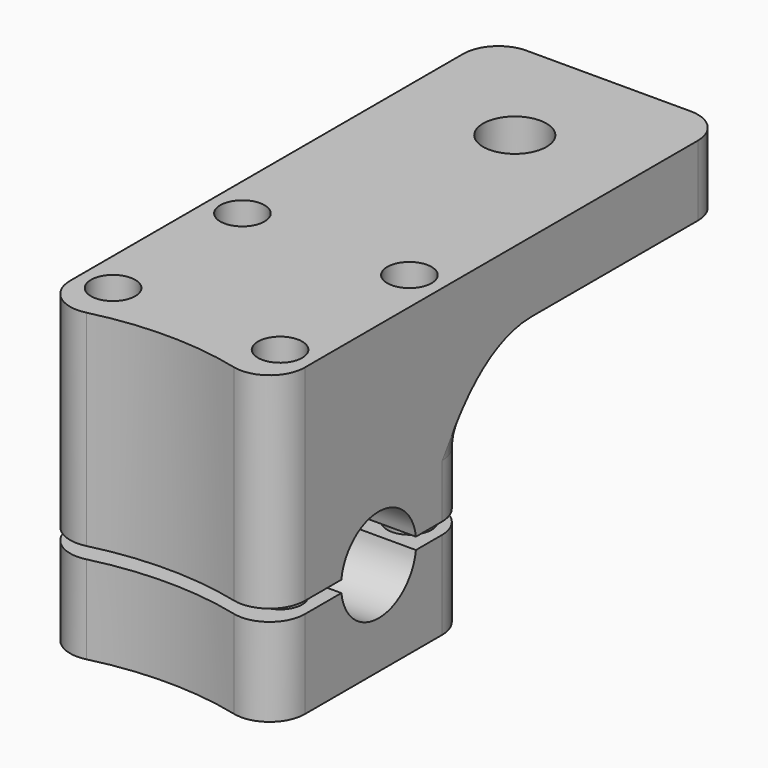
from build123d import *

# Parameters (mm, degrees)
F0_W         = 20
F0_H         = 22.7722101178
F0_R         = 1.8861050589
F0_H_2       = 26.2277898822
F0_R_2       = 2.7
F1_DEPTH     = 6
F2_DEPTH     = 20
F4_DEPTH     = 20.001
F6_DEPTH     = 20
F7_DEPTH     = 26.001
F8_R         = 3
F9_T2_ANGLE  = 25.7767353783
F9_T6_ANGLE  = 359.64
F9_T11_ANGLE = 359.64
F10_DEPTH    = 20.0010001


# Not quite as in the source:
# - a fillet or chamfer that OpenCascade refuses, or shapes differently, is made with other operations: its cross-section is extruded or revolved along the edge and cut away or added


with BuildPart() as f1:
    # F0 (on Top) → F1 (new body)
    with BuildSketch(Plane.XY):
        with Locations((0, -13.1138949411)):
            Rectangle(F0_W, F0_H)
        with Locations((-7.1138949411, -19.3861050589)):
            Circle(F0_R, mode=Mode.SUBTRACT)
        with Locations((-7.1138949411, -5.6138949411)):
            Circle(F0_R, mode=Mode.SUBTRACT)
        with Locations((7.1138949411, -19.3861050589)):
            Circle(F0_R, mode=Mode.SUBTRACT)
        with Locations((7.1138949411, -5.6138949411)):
            Circle(F0_R, mode=Mode.SUBTRACT)
        with Locations((0, 11.3861050589)):
            Rectangle(F0_W, F0_H_2)
        with Locations((0, 14.5)):
            Circle(F0_R_2, mode=Mode.SUBTRACT)
    extrude(amount=F1_DEPTH)

    # F0 (on Top) → F2 (join)
    with BuildSketch(Plane.XY):
        with Locations((0, -13.1138949411)):
            Rectangle(F0_W, F0_H)
        with Locations((-7.1138949411, -19.3861050589)):
            Circle(F0_R, mode=Mode.SUBTRACT)
        with Locations((-7.1138949411, -5.6138949411)):
            Circle(F0_R, mode=Mode.SUBTRACT)
        with Locations((7.1138949411, -19.3861050589)):
            Circle(F0_R, mode=Mode.SUBTRACT)
        with Locations((7.1138949411, -5.6138949411)):
            Circle(F0_R, mode=Mode.SUBTRACT)
    extrude(amount=-F2_DEPTH)

    # F3 (on face) → F4 (cut, through all)
    with BuildSketch(Plane.YZ.offset(10)):
        with BuildLine():
            Line((-16.5, -12), (-8.5, -12))
            ThreePointArc((-8.5, -12), (-8.5078509631, -11.7495083498), (-8.5313730334, -11.5))
            Line((-8.5313730334, -11.5), (-16.4686269666, -11.5))
            ThreePointArc((-16.4686269666, -11.5), (-16.4921490369, -11.7495083498), (-16.5, -12))
        make_face()
        with BuildLine():
            ThreePointArc((-8.5313730334, -12.5), (-8.5078509631, -12.2504916502), (-8.5, -12))
            Line((-8.5, -12), (-16.5, -12))
            ThreePointArc((-16.5, -12), (-16.4921490369, -12.2504916502), (-16.4686269666, -12.5))
            Line((-16.4686269666, -12.5), (-8.5313730334, -12.5))
        make_face()
        with BuildLine():
            Line((-16.4686269666, -11.5), (-8.5313730334, -11.5))
            ThreePointArc((-8.5313730334, -11.5), (-12.5, -8), (-16.4686269666, -11.5))
        make_face()
        with BuildLine():
            ThreePointArc((-16.4686269666, -12.5), (-12.5, -16), (-8.5313730334, -12.5))
            Line((-8.5313730334, -12.5), (-16.4686269666, -12.5))
        make_face()
    extrude(amount=-F4_DEPTH, mode=Mode.SUBTRACT)

    # F5 (on face) → F6 (cut, through all)
    with BuildSketch(Plane(origin=(0, 0, -20), x_dir=(1, 0, 0), z_dir=(0, 0, -1))):
        with BuildLine():
            Line((-10, 1.7277898822), (10, 1.7277898822))
            ThreePointArc((10, 1.7277898822), (0, 3.5477721311), (-10, 1.7277898822))
        make_face()
    extrude(amount=-F6_DEPTH, mode=Mode.SUBTRACT)

    # F5 (on face) → F7 (cut, through all)
    with BuildSketch(Plane(origin=(0, 0, -20), x_dir=(1, 0, 0), z_dir=(0, 0, -1))):
        with BuildLine():
            ThreePointArc((-10, 24.5), (0, 22.5), (10, 24.5))
            Line((10, 24.5), (-10, 24.5))
        make_face()
    extrude(amount=-F7_DEPTH, mode=Mode.SUBTRACT)

    # F8
    f8_edges = [f1.edges().sort_by_distance(p)[0] for p in [
        (-10, 24.5, 3),
        (10, 24.5, 3),
        (10, -24.5, -7),
        (-10, -24.5, -7),
        (-10, -1.72779, -10),
        (10, -1.72779, -10),
    ]]
    fillet(f8_edges, radius=F8_R)

    # F9: fillet of radius 7 on 1 edges, made by hand

    # F9_s1 → F9_t2 (revolve)
    with BuildSketch(Plane(origin=(5.3999454097, 1.2355988362, 0), x_dir=(0, 0, 1), z_dir=(0.9748064988, 0.2230522133, 0))):
        with BuildLine():
            ThreePointArc((0.0004, -2.8275125891), (-2.0502525317, 2.1232005646), (-7.0009656854, 4.1738530963))
            Line((-7.0009656854, 4.1738530963), (-7.0009656854, 4.8739896648))
            ThreePointArc((-7.0009656854, 4.8739896648), (-3.5004828427, 4.8735896648), (0, 4.8735896648))
            Line((0, 4.8735896648), (0.7001365685, 4.1734530963))
            ThreePointArc((0.7001365685, 4.1734530963), (0.7001365685, 0.6729702536), (0.7005365685, -2.8275125891))
            Line((0.7005365685, -2.8275125891), (0.0004, -2.8275125891))
        make_face()
    revolve(axis=Axis((0, 24.8350144179, 0), (0, 0, -1)), revolution_arc=F9_T2_ANGLE)


with BuildPart() as f9_tool4:
    # F9_s5 → F9_t6 (revolve)
    with BuildSketch(Plane(origin=(5.3999454097, 1.2355988362, 0), x_dir=(0, 0, 1), z_dir=(-0.9748064988, -0.2230522133, 0))):
        with BuildLine():
            ThreePointArc((0.0004, 2.8275125891), (-2.0502525317, -2.1232005646), (-7.0009656854, -4.1738530963))
            Line((-7.0009656854, -4.1738530963), (-7.0009656854, -4.8739896648))
            ThreePointArc((-7.0009656854, -4.8739896648), (-3.5004828427, -4.8735896648), (0, -4.8735896648))
            Line((0, -4.8735896648), (0.7001365685, -4.1734530963))
            ThreePointArc((0.7001365685, -4.1734530963), (0.7001365685, -0.6729702536), (0.7005365685, 2.8275125891))
            Line((0.7005365685, 2.8275125891), (0.0004, 2.8275125891))
        make_face()
    revolve(axis=Axis((7, -5.757129861, 0), (0, 0, -1)), revolution_arc=F9_T6_ANGLE)

    split(bisect_by=Plane.YZ.offset(10), keep=Keep.BOTTOM)


with BuildPart() as f1_1:
    add(f1.part)

    # F9_t3: union F9_tool4
    add(f9_tool4.part)


with BuildPart() as f9_tool9:
    # F9_s10 → F9_t11 (revolve)
    with BuildSketch(Plane(origin=(-5.348096652, 1.2591487889, 0), x_dir=(0, 0, 1), z_dir=(-0.9733857878, 0.22917266, 0))):
        with BuildLine():
            ThreePointArc((0.0004, 2.79284868), (-2.0502525317, -2.1578644738), (-7.0009656854, -4.2085170055))
            Line((-7.0009656854, -4.2085170055), (-7.0009656854, -4.908653574))
            ThreePointArc((-7.0009656854, -4.908653574), (-3.5004828427, -4.908253574), (0, -4.908253574))
            Line((0, -4.908253574), (0.7001365685, -4.2081170055))
            ThreePointArc((0.7001365685, -4.2081170055), (0.7001365685, -0.7076341628), (0.7005365685, 2.79284868))
            Line((0.7005365685, 2.79284868), (0.0004, 2.79284868))
        make_face()
    revolve(axis=Axis((-7, -5.757129861, 0), (0, 0, -1)), revolution_arc=F9_T11_ANGLE)

    split(bisect_by=Plane.YZ.offset(-10), keep=Keep.TOP)


with BuildPart() as f1_2:
    add(f1_1.part)

    # F9_t8: union F9_tool9
    add(f9_tool9.part)

    # F3 (on face) → F10 (cut, through all)
    with BuildSketch(Plane.YZ.offset(10)):
        with BuildLine():
            ThreePointArc((-16.4686269666, -12.5), (-16.4921490369, -12.2504916502), (-16.5, -12))
            Line((-16.5, -12), (-24.5, -12))
            Line((-24.5, -12), (-24.5, -12.5))
            Line((-24.5, -12.5), (-16.4686269666, -12.5))
        make_face()
        with BuildLine():
            Line((-24.5, -12), (-16.5, -12))
            ThreePointArc((-16.5, -12), (-16.4921490369, -11.7495083498), (-16.4686269666, -11.5))
            Line((-16.4686269666, -11.5), (-24.5, -11.5))
            Line((-24.5, -11.5), (-24.5, -12))
        make_face()
        with BuildLine():
            ThreePointArc((-8.5313730334, -12.5), (-8.5078509631, -12.2504916502), (-8.5, -12))
            Line((-8.5, -12), (-16.5, -12))
            ThreePointArc((-16.5, -12), (-16.4921490369, -12.2504916502), (-16.4686269666, -12.5))
            Line((-16.4686269666, -12.5), (-8.5313730334, -12.5))
        make_face()
        with BuildLine():
            Line((-16.5, -12), (-8.5, -12))
            ThreePointArc((-8.5, -12), (-8.5078509631, -11.7495083498), (-8.5313730334, -11.5))
            Line((-8.5313730334, -11.5), (-16.4686269666, -11.5))
            ThreePointArc((-16.4686269666, -11.5), (-16.4921490369, -11.7495083498), (-16.5, -12))
        make_face()
        with BuildLine():
            ThreePointArc((-8.5313730334, -11.5), (-8.5078509631, -11.7495083498), (-8.5, -12))
            Line((-8.5, -12), (-1.7277898822, -12))
            Line((-1.7277898822, -12), (-1.7277898822, -11.5))
            Line((-1.7277898822, -11.5), (-8.5313730334, -11.5))
        make_face()
        with BuildLine():
            Line((-1.7277898822, -12), (-8.5, -12))
            ThreePointArc((-8.5, -12), (-8.5078509631, -12.2504916502), (-8.5313730334, -12.5))
            Line((-8.5313730334, -12.5), (-1.7277898822, -12.5))
            Line((-1.7277898822, -12.5), (-1.7277898822, -12))
        make_face()
    extrude(amount=-F10_DEPTH, mode=Mode.SUBTRACT)


solid = f1_2.part
